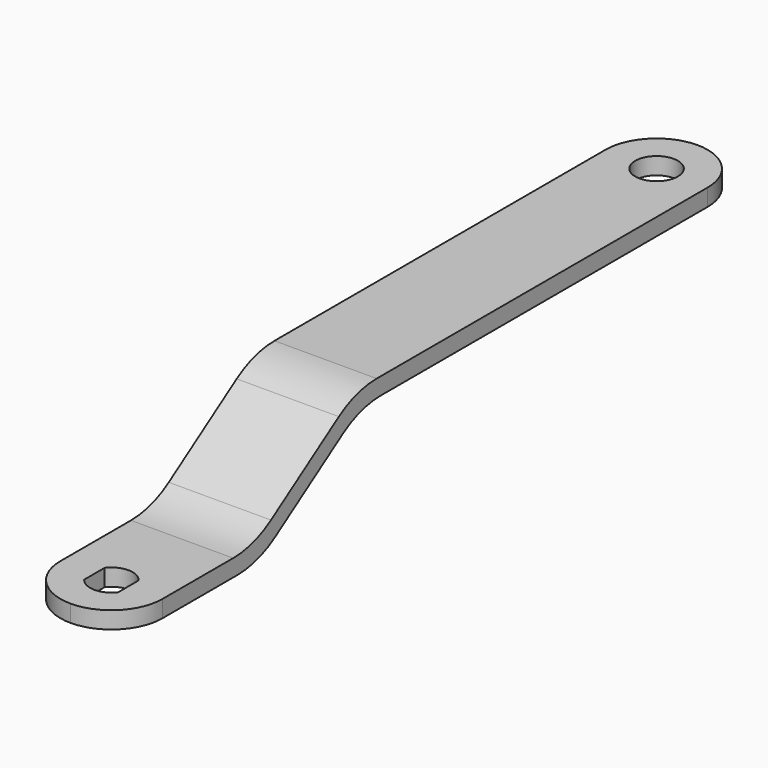
from build123d import *

# Parameters (mm, degrees)
F1_W     = 12
F1_H     = 2
F3_R     = 10
F5_DEPTH = 12.001
F6_R     = 2.5
F7_DEPTH = 12.001
F8_R     = 5.99999
F9_R     = 5.99999


# Not quite as in the source:
# - a fillet or chamfer is up to 0.001 mm smaller than in the source, because OpenCascade refuses the exact size


with BuildPart() as f2:
    # F2: sweep along a path in F0
    with BuildLine(Plane.YZ) as f2_path:
        Line((0, 0), (20, 0))
        Line((20, 0), (35, 10))
        Line((35, 10), (92, 10))
    # F1 (on Front) → F2 (sweep)
    with BuildSketch(Plane.XZ):
        with Locations((0, 1)):
            Rectangle(F1_W, F1_H)
    sweep(path=f2_path.line, transition=Transition.RIGHT)

    # F3
    f3_edges = [f2.edges().sort_by_distance(p)[0] for p in [
        (0, 19.394449, 2),
        (0, 34.394449, 12),
        (0, 35, 10),
        (0, 20, 0),
    ]]
    fillet(f3_edges, radius=F3_R)

    # F4 (on Top) → F5 (cut, through all)
    with BuildSketch(Plane.XY):
        with BuildLine():
            Line((2, 4.5), (2, 7.5))
            ThreePointArc((2, 7.5), (0, 8.5), (-2, 7.5))
            Line((-2, 7.5), (-2, 4.5))
            ThreePointArc((-2, 4.5), (0, 3.5), (2, 4.5))
        make_face()
    extrude(amount=F5_DEPTH, mode=Mode.SUBTRACT)

    # F6 (on Top) → F7 (cut, through all)
    with BuildSketch(Plane.XY):
        with Locations((0, 86)):
            Circle(F6_R)
    extrude(amount=F7_DEPTH, mode=Mode.SUBTRACT)

    # F8 (radius 6 in the source; OpenCascade refuses exactly that, so slightly less here)
    f8_edges = [f2.edges().sort_by_distance(p)[0] for p in [
        (-6, 0, 1),
        (6, 0, 1),
    ]]
    fillet(f8_edges, radius=F8_R)

    # F9 (radius 6 in the source; OpenCascade refuses exactly that, so slightly less here)
    f9_edges = [f2.edges().sort_by_distance(p)[0] for p in [
        (6, 92, 11),
        (-6, 92, 11),
    ]]
    fillet(f9_edges, radius=F9_R)


solid = f2.part
